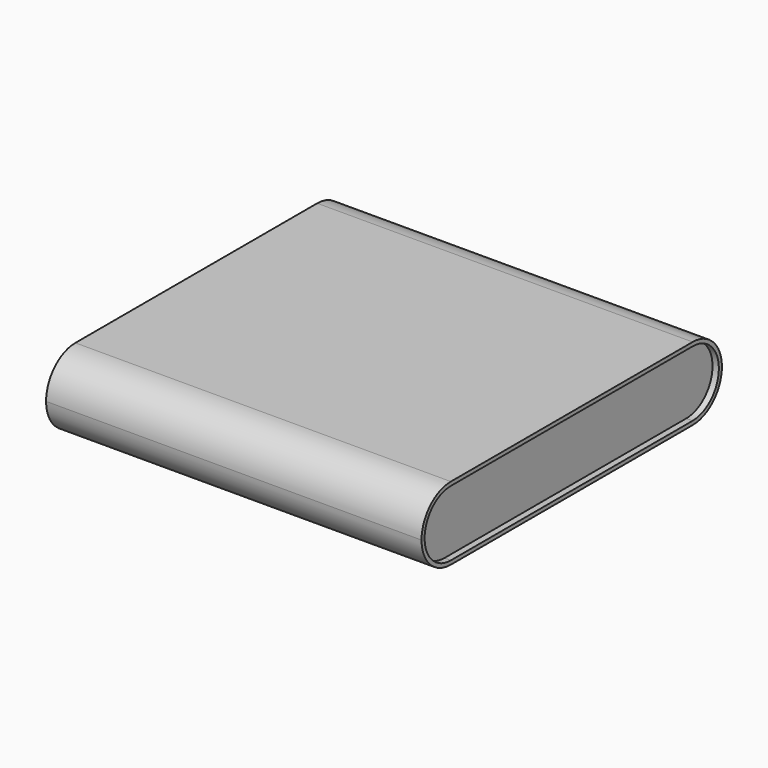
from build123d import *

# Parameters (mm, degrees)
F0_W     = 59
F0_H     = 59
F1_DEPTH = 11.5
F2_R     = 5.74999
F4_DEPTH = 1
F6_DEPTH = 1
F8_DEPTH = 1


# Not quite as in the source:
# - a fillet or chamfer is up to 0.001 mm smaller than in the source, because OpenCascade refuses the exact size


with BuildPart() as f1:
    # F0 (on Top) → F1 (new body)
    with BuildSketch(Plane.XY):
        with Locations((29.5, -29.5)):
            Rectangle(F0_W, F0_H)
    extrude(amount=F1_DEPTH)

    # F2 (radius 5.75 in the source; OpenCascade refuses exactly that, so slightly less here)
    f2_edges = [f1.edges().sort_by_distance(p)[0] for p in [
        (29.5, -59, 11.5),
        (29.5, -59, 0),
        (29.5, 0, 11.5),
        (29.5, 0, 0),
    ]]
    fillet(f2_edges, radius=F2_R)

    # F3 (on face) → F4 (cut)
    with BuildSketch(Plane.YZ.offset(59)):
        with BuildLine():
            ThreePointArc((-5.75, 0.5999998897), (-0.5999998897, 5.75), (-5.75, 10.9000001103))
            Line((-5.75, 10.9000001103), (-53.25, 10.9000001103))
            ThreePointArc((-53.25, 10.9000001103), (-58.4000001103, 5.75), (-53.25, 0.5999998897))
            Line((-53.25, 0.5999998897), (-5.75, 0.5999998897))
        make_face()
    extrude(amount=-F4_DEPTH, mode=Mode.SUBTRACT)

    # F5 (on face) → F6 (cut)
    with BuildSketch(Plane(origin=(0, 0, 0), x_dir=(0, -1, 0), z_dir=(-1, 0, 0))):
        with BuildLine():
            Line((53.25, 10.9), (5.75, 10.9))
            ThreePointArc((5.75, 10.9), (0.6, 5.75), (5.75, 0.6))
            Line((5.75, 0.6), (53.25, 0.6))
            ThreePointArc((53.25, 0.6), (58.4, 5.75), (53.25, 10.9))
        make_face()
    extrude(amount=-F6_DEPTH, mode=Mode.SUBTRACT)


with BuildPart() as f8:
    # F7 (on face) → F8 (new body)
    with BuildSketch(Plane(origin=(0, 0, 0), x_dir=(1, 0, 0), z_dir=(0, 0, -1))):
        Polygon((57.5, 39.5), (50.5, 39.5), (50.5, 19.5), (57.5, 19.5), (57.5, 29.5), align=None)
    extrude(amount=F8_DEPTH)


solid = Compound([f1.part, f8.part])
